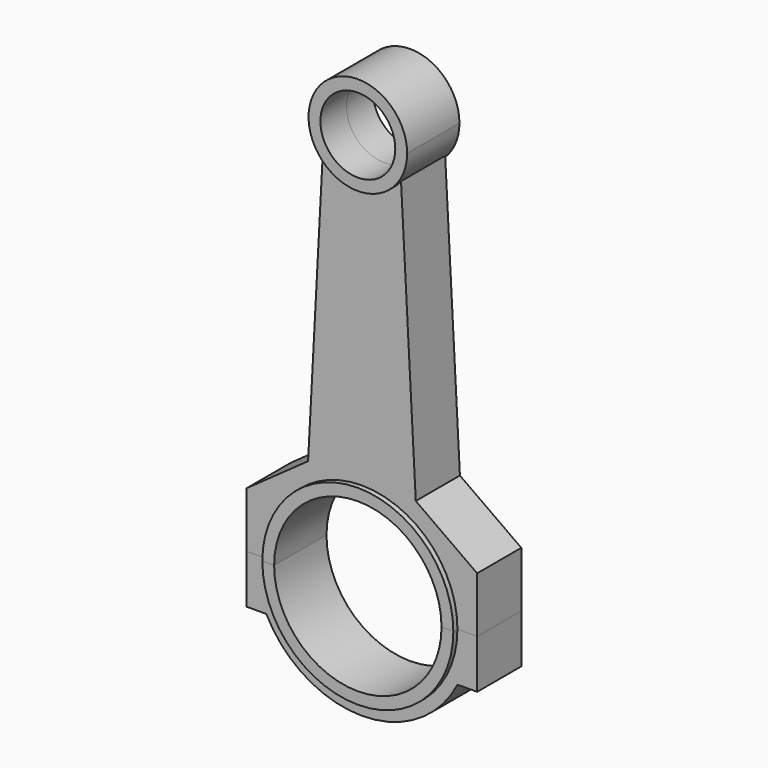
from build123d import *

# Parameters (mm, degrees)
F1_DEPTH = 10.541
F2_DEPTH = 8.89
F3_DEPTH = 10.541
F4_DEPTH = 8.89
F0_R     = 12.065
F5_DEPTH = 10.541


with BuildPart() as f1:
    # F0 (on Front) → F1 (new body, symmetric)
    with BuildSketch(Plane.XZ):
        with BuildLine():
            ThreePointArc((-26.9621, -63.1996413046), (0, -36.2375413046), (26.9621, -63.1996413046))
            Line((26.9621, -63.1996413046), (30.7721, -63.1996413046))
            ThreePointArc((30.7721, -63.1996413046), (0, -32.4275413046), (-30.7721, -63.1996413046))
            Line((-30.7721, -63.1996413046), (-26.9621, -63.1996413046))
        make_face()
    extrude(amount=F1_DEPTH, both=True)

    # F0 (on Front) → F2 (join, symmetric)
    with BuildSketch(Plane.XZ):
        with BuildLine():
            ThreePointArc((-30.7721, -63.1996413046), (0, -32.4275413046), (30.7721, -63.1996413046))
            Line((30.7721, -63.1996413046), (37.1221, -63.1996413046))
            Line((37.1221, -63.1996413046), (37.1221, -45.2870428562))
            Line((37.1221, -45.2870428562), (17.3492934555, -31.2083195895))
            Line((17.3492934555, -31.2083195895), (12.597056389, 57.9496239752))
            ThreePointArc((12.597056389, 57.9496239752), (0, 51.7353586954), (-12.597056389, 57.9496239752))
            Line((-12.597056389, 57.9496239752), (-17.3492934555, -31.2083195895))
            Line((-17.3492934555, -31.2083195895), (-37.1221, -45.2870428562))
            Line((-37.1221, -45.2870428562), (-37.1221, -63.1996413046))
            Line((-37.1221, -63.1996413046), (-30.7721, -63.1996413046))
        make_face()
    extrude(amount=F2_DEPTH, both=True)

    # F0 (on Front) → F5 (join, symmetric)
    with BuildSketch(Plane.XZ):
        with BuildLine():
            ThreePointArc((-12.597056389, 57.9496239752), (0, 51.7353586954), (12.597056389, 57.9496239752))
            ThreePointArc((12.597056389, 57.9496239752), (15.0331948563, 62.5095080396), (15.875, 67.6103586954))
            ThreePointArc((15.875, 67.6103586954), (-5.1008506558, 82.6435535517), (-12.597056389, 57.9496239752))
        make_face()
        with Locations((0, 67.6103586954)):
            Circle(F0_R, mode=Mode.SUBTRACT)
    extrude(amount=F5_DEPTH, both=True)


with BuildPart() as f3:
    # F0 (on Front) → F3 (new body, symmetric)
    with BuildSketch(Plane.XZ):
        with BuildLine():
            Line((30.7721, -63.1996413046), (26.9621, -63.1996413046))
            ThreePointArc((26.9621, -63.1996413046), (0, -90.1617413046), (-26.9621, -63.1996413046))
            Line((-26.9621, -63.1996413046), (-30.7721, -63.1996413046))
            ThreePointArc((-30.7721, -63.1996413046), (0, -93.9717413046), (30.7721, -63.1996413046))
        make_face()
    extrude(amount=F3_DEPTH, both=True)

    # F0 (on Front) → F4 (join, symmetric)
    with BuildSketch(Plane.XZ):
        with BuildLine():
            Line((37.1221, -63.1996413046), (30.7721, -63.1996413046))
            ThreePointArc((30.7721, -63.1996413046), (0, -93.9717413046), (-30.7721, -63.1996413046))
            Line((-30.7721, -63.1996413046), (-37.1221, -63.1996413046))
            Line((-37.1221, -63.1996413046), (-37.1221, -78.9195522666))
            Line((-37.1221, -78.9195522666), (-30.8026953327, -78.9195522666))
            ThreePointArc((-30.8026953327, -78.9195522666), (0, -97.7817413046), (30.8026953327, -78.9195522666))
            Line((30.8026953327, -78.9195522666), (37.1221, -78.9195522666))
            Line((37.1221, -78.9195522666), (37.1221, -63.1996413046))
        make_face()
    extrude(amount=F4_DEPTH, both=True)


solid = Compound([f1.part, f3.part])
